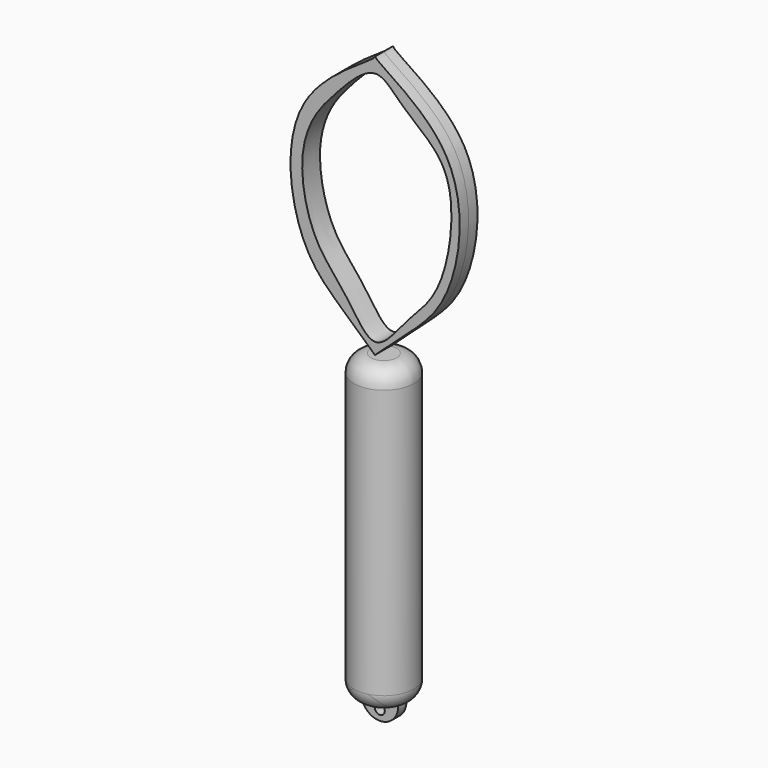
from build123d import *

# Parameters (mm, degrees)
F0_R         = 8.89
F1_DEPTH     = 89.916
F3_DEPTH     = 1.524
F4_R         = 1.4939086428
F5_DEPTH     = 10.415
F7_DEPTH     = 3.302
F9_DEPTH     = 12.193
F10_S5_R     = 5.4694928486
F10_T6_DEPTH = 14


# Not quite as in the source:
# - a fillet or chamfer that OpenCascade refuses, or shapes differently, is made with other operations: its cross-section is extruded or revolved along the edge and cut away or added


with BuildPart() as f1:
    # F0 (on Top) → F1 (new body)
    with BuildSketch(Plane.XY):
        Circle(F0_R)
    extrude(amount=F1_DEPTH)

    # F2 (on Front) → F3 (join, symmetric)
    with BuildSketch(Plane.XZ):
        with BuildLine():
            Line((5.3248568295, 1.2495006065), (-5.4186682252, 0.7438996476))
            ThreePointArc((-5.4186682252, 0.7438996476), (0.2571152016, -5.4634461463), (5.3248568295, 1.2495006065))
        make_face()
    extrude(amount=F3_DEPTH, both=True)

    # F4 (on face) → F5 (cut, through all)
    with BuildSketch(Plane.XZ.offset(1.524)):
        with Locations((0, -2.4195204023)):
            Circle(F4_R)
    extrude(amount=-F5_DEPTH, mode=Mode.SUBTRACT)

    # F10: fillet of radius 5.08 on 3 edges, made by hand


with BuildPart() as f7:
    # F6 (on Front) → F7 (new body, symmetric)
    with BuildSketch(Plane.XZ):
        with BuildLine():
            add(Edge.make_bspline(
                [(0, 90.7432958488), (-3.6411630759, 94.0368409573), (-11.2084804517, 100.8817145889), (-23.9517565636, 112.7489507769), (-29.3104718471, 153.1175855958), (-0.670400138, 167.0245086595), (0.0705790091, 168.6812087159), (0.0849867676, 168.7365486509)],
                knots=[0, 0, 0, 0, 0.1916614812, 0.3983241692, 0.7016663836, 0.9617657107, 0.9715620142, 0.9715620142, 0.9715620142, 0.9715620142], degree=3))
            add(Edge.make_bspline(
                [(0, 90.7432958488), (3.6483321632, 94.0288978262), (11.2305488332, 100.8572634922), (23.9996573521, 112.6966996459), (29.446336641, 153.0535601699), (0.8366407727, 167.0228664849), (0.0992738876, 168.681177448), (0.0849867676, 168.7365486509)],
                knots=[0, 0, 0, 0, 0.1916614812, 0.3983241692, 0.7016663836, 0.9617657107, 0.9715620142, 0.9715620142, 0.9715620142, 0.9715620142], degree=3))
        make_face()
    extrude(amount=F7_DEPTH, both=True)

    # F8 (on face) → F9 (cut, through all)
    with BuildSketch(Plane.XZ.offset(3.302)):
        with BuildLine():
            add(Edge.make_bspline(
                [(0, 94.2149311304), (2.8065520098, 94.1239459522), (8.7296647114, 102.4297246395), (15.3171707229, 108.4672293564), (20.3807405485, 116.9635877784), (23.5112168499, 132.4815508586), (21.6544342813, 148.8669118709), (7.6781914455, 157.8150938857), (0.2236564599, 167.8824485493), (-11.8962797808, 155.114358939), (-18.7050108308, 147.2261937135), (-23.0355139647, 134.3181025818), (-18.8737269323, 114.2565687243), (-8.4728537436, 104.5548865414), (-2.905504055, 94.3091242197), (0, 94.2149311304)],
                knots=[0, 0, 0, 0, 0.0715081172, 0.1376819399, 0.2026320222, 0.2869937301, 0.3707675266, 0.4562551298, 0.5216900081, 0.6017803775, 0.6729002391, 0.749053263, 0.84247562, 0.9259706844, 1, 1, 1, 1], degree=3))
        make_face()
    extrude(amount=-F9_DEPTH, mode=Mode.SUBTRACT)


with BuildPart() as f10_tool2:
    # F10_s3 → F10_t4 (revolve)
    with BuildSketch(Plane.XZ):
        with BuildLine():
            ThreePointArc((8.89, 5.08), (7.4021024484, 1.4878975516), (3.81, 0))
            Line((3.81, 0), (8.89, 0))
            Line((8.89, 0), (8.89, 5.08))
        make_face()
    revolve(axis=Axis((0, 0, 0), (0, 0, 1)))

    # F10_s5 → F10_t6 (cut, symmetric)
    with BuildSketch(Plane.XZ):
        Circle(F10_S5_R)
    extrude(amount=F10_T6_DEPTH, both=True, mode=Mode.SUBTRACT)


with BuildPart() as f1_1:
    add(f1.part)

    # F10_t1: cut F10_tool2
    add(f10_tool2.part, mode=Mode.SUBTRACT)


with BuildPart() as f10_tool8:
    # F10_s9 → F10_t10 (revolve)
    with BuildSketch(Plane.XZ):
        with BuildLine():
            ThreePointArc((8.89, 5.08), (7.4021024484, 1.4878975516), (3.81, 0))
            Line((3.81, 0), (8.89, 0))
            Line((8.89, 0), (8.89, 5.08))
        make_face()
    revolve(axis=Axis((0, 0, 0), (0, 0, 1)))

    split(bisect_by=Plane.XZ.offset(-1.524), keep=Keep.BOTTOM)


with BuildPart() as f1_2:
    add(f1_1.part)

    # F10_t7: cut F10_tool8
    add(f10_tool8.part, mode=Mode.SUBTRACT)


with BuildPart() as f10_tool13:
    # F10_s14 → F10_t15 (revolve)
    with BuildSketch(Plane.XZ):
        with BuildLine():
            ThreePointArc((8.89, 5.08), (7.4021024484, 1.4878975516), (3.81, 0))
            Line((3.81, 0), (8.89, 0))
            Line((8.89, 0), (8.89, 5.08))
        make_face()
    revolve(axis=Axis((0, 0, 0), (0, 0, 1)))

    split(bisect_by=Plane.XZ.offset(1.524), keep=Keep.TOP)


with BuildPart() as f1_3:
    add(f1_2.part)

    # F10_t12: cut F10_tool13
    add(f10_tool13.part, mode=Mode.SUBTRACT)

    # F10_s17 → F10_t18 (revolve, cut)
    with BuildSketch(Plane.XZ):
        with BuildLine():
            ThreePointArc((8.89, 84.836), (7.4021024484, 88.4281024484), (3.81, 89.916))
            Line((3.81, 89.916), (8.89, 89.916))
            Line((8.89, 89.916), (8.89, 84.836))
        make_face()
    revolve(axis=Axis((0, 0, 89.916), (0, 0, 1)), mode=Mode.SUBTRACT)


solid = Compound([f7.part, f1_3.part])
